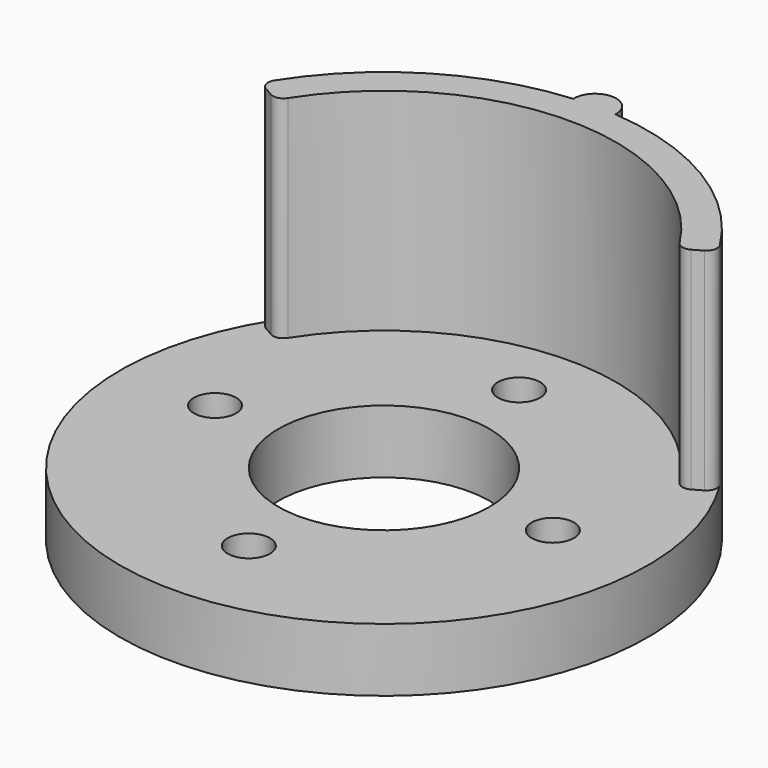
from build123d import *

# Parameters (mm, degrees)
F0_R            = 317.5
F0_R_2          = 127
F1_DEPTH        = 76.2
F3_DEPTH        = 254
F4_R            = 12.7
F6_DEPTH        = 330.2
F7_R            = 25.4
F8_DEPTH        = 76.201
F8_COPIES_COUNT = 4


# Not quite as in the source:
# - a pattern or mirror of a feature is missing from the dataset's text; its kind, count and spacing are read off the source's solid


with BuildPart() as f1:
    # F0 (on Top) → F1 (new body)
    with BuildSketch(Plane.XY):
        Circle(F0_R)
        Circle(F0_R_2, mode=Mode.SUBTRACT)
    extrude(amount=F1_DEPTH)

    # F2 (on face) → F3 (join)
    with BuildSketch(Plane.XY.offset(76.2)):
        with BuildLine():
            ThreePointArc((-241.9674978174, 139.7), (0, 279.4), (241.9674978174, 139.7))
            Line((241.9674978174, 139.7), (274.9630657016, 158.75))
            ThreePointArc((274.9630657016, 158.75), (0, 317.5), (-274.9630657016, 158.75))
            Line((-274.9630657016, 158.75), (-241.9674978174, 139.7))
        make_face()
    extrude(amount=F3_DEPTH)

    # F4
    f4_edges = [f1.edges().sort_by_distance(p)[0] for p in [
        (-274.963066, 158.75, 203.2),
        (-241.967498, 139.7, 203.2),
        (241.967498, 139.7, 203.2),
        (274.963066, 158.75, 203.2),
    ]]
    fillet(f4_edges, radius=F4_R)

    # F5 (on face) → F6 (join, through all)
    with BuildSketch(Plane.XY.offset(330.2)):
        with BuildLine():
            ThreePointArc((25.3796718655, 316.484), (25.3949174579, 316.9918983288), (25.4, 317.5))
            ThreePointArc((25.4, 317.5), (-0.5081016712, 342.8949174579), (-25.3796718655, 316.484))
            ThreePointArc((-25.3796718655, 316.484), (0, 317.5), (25.3796718655, 316.484))
        make_face()
        with BuildLine():
            ThreePointArc((25.3796718655, 316.484), (0, 317.5), (-25.3796718655, 316.484))
            ThreePointArc((-25.3796718655, 316.484), (0, 292.1), (25.3796718655, 316.484))
        make_face()
    extrude(amount=-F6_DEPTH)

    # F7 (on face) → F8 (cut, through all)
    with BuildSketch(Plane.XY.offset(76.2)):
        with Locations((-203.2, 0)):
            Circle(F7_R)
    f8 = extrude(amount=-F8_DEPTH, mode=Mode.SUBTRACT)

    # F8_copies: F8 ×4 about axis
    f8_copies_axis = Axis((0, 0, 0), (0, 0, 1))
    for i in range(1, F8_COPIES_COUNT):
        add(f8.rotate(f8_copies_axis, i * 360 / F8_COPIES_COUNT), mode=Mode.SUBTRACT)


solid = f1.part
